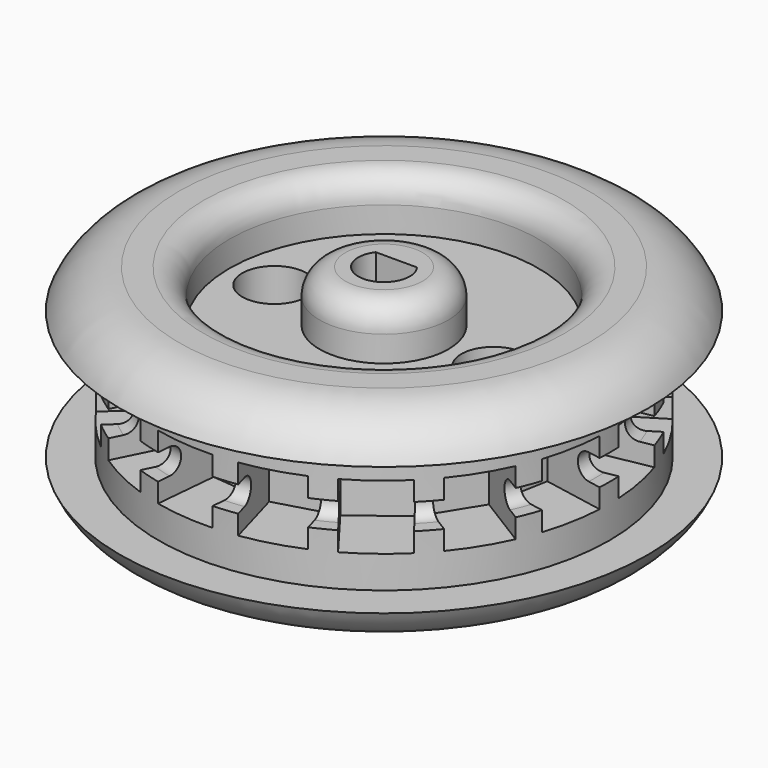
from build123d import *

# Parameters (mm, degrees)
F0_R      = 17.5
F1_DEPTH  = 10
F8_R      = 20.5
F8_R_2    = 17.5
F6_R      = 17.5
F9_DEPTH  = 3
F7_R      = 17.5
F10_R     = 20.5
F10_R_2   = 17.5
F11_DEPTH = 3
F14_DEPTH = 16.001
F15_R     = 4
F16_DEPTH = 5
F17_R     = 12
F17_R_2   = 8.5
F17_R_3   = 5
F18_DEPTH = 4
F19_R     = 2
F3_W      = 5
F3_H      = 4.6
F20_DEPTH = 2.5
F22_R     = 2.5
F23_DEPTH = 13


# Not quite as in the source:
# - a fillet or chamfer that OpenCascade refuses, or shapes differently, is made with other operations: its cross-section is extruded or revolved along the edge and cut away or added


with BuildPart() as f1:
    # F0 (on Top) → F1 (new body)
    with BuildSketch(Plane.XY):
        Circle(F0_R)
    extrude(amount=F1_DEPTH)

    # F8 (on face) + F6 (on face) → F9 (join)
    with BuildSketch(Plane.XY.offset(10)):
        Circle(F8_R)
        Circle(F8_R_2, mode=Mode.SUBTRACT)
    with BuildSketch(Plane.XY.offset(10)):
        Circle(F6_R)
    extrude(amount=F9_DEPTH)

    # F7 (on face) + F10 (on face) → F11 (join)
    with BuildSketch(Plane(origin=(0, 0, 0), x_dir=(1, 0, 0), z_dir=(0, 0, -1))):
        Circle(F7_R)
    with BuildSketch(Plane(origin=(0, 0, 0), x_dir=(1, 0, 0), z_dir=(0, 0, -1))):
        Circle(F10_R)
        Circle(F10_R_2, mode=Mode.SUBTRACT)
    extrude(amount=F11_DEPTH)

    # F12: fillet of radius 5 on 2 edges, made by hand

    # F12_s1 → F12_t2 (revolve, cut)
    with BuildSketch(Plane.XZ):
        with BuildLine():
            ThreePointArc((20.5, 0), (18.6560370926, -2.1833001327), (15.917424305, -3))
            Line((15.917424305, -3), (20.5, -3))
            Line((20.5, -3), (20.5, 0))
        make_face()
    revolve(axis=Axis((0, 0, -3), (0, 0, -1)), mode=Mode.SUBTRACT)

    # F12_s3 → F12_t4 (revolve, cut)
    with BuildSketch(Plane.XZ):
        with BuildLine():
            ThreePointArc((20.5, 10), (18.6560370926, 12.1833001327), (15.917424305, 13))
            Line((15.917424305, 13), (20.5, 13))
            Line((20.5, 13), (20.5, 10))
        make_face()
    revolve(axis=Axis((0, 0, 13), (0, 0, 1)), mode=Mode.SUBTRACT)

    # F13 (on face) → F14 (cut, through all)
    with BuildSketch(Plane.XY.offset(13)):
        with BuildLine():
            ThreePointArc((-1.6, 1.2), (-0.632455532, -1.8973665961), (2, 0))
            ThreePointArc((2, 0), (1.8973665961, 0.632455532), (1.6, 1.2))
            Line((1.6, 1.2), (-1.6, 1.2))
        make_face()
    extrude(amount=-F14_DEPTH, mode=Mode.SUBTRACT)

    # F15 (on face) → F16 (cut)
    with BuildSketch(Plane(origin=(0, 0, -3), x_dir=(1, 0, 0), z_dir=(0, 0, -1))):
        Circle(F15_R)
        with BuildLine():
            ThreePointArc((2, 0), (1.8973665961, -0.632455532), (1.6, -1.2))
            Line((1.6, -1.2), (-1.6, -1.2))
            ThreePointArc((-1.6, -1.2), (-0.632455532, 1.8973665961), (2, 0))
        make_face(mode=Mode.SUBTRACT)
    extrude(amount=-F16_DEPTH, mode=Mode.SUBTRACT)

    # F17 (on face) → F18 (cut)
    with BuildSketch(Plane.XY.offset(13)):
        Circle(F17_R)
        Circle(F17_R_2, mode=Mode.SUBTRACT)
        Circle(F17_R_2)
        Circle(F17_R_3, mode=Mode.SUBTRACT)
    extrude(amount=-F18_DEPTH, mode=Mode.SUBTRACT)

    # F19
    f19_edges = [f1.edges().sort_by_distance(p)[0] for p in [
        (-12, 0, 13),
        (-5, 0, 13),
    ]]
    fillet(f19_edges, radius=F19_R)

    # F3 (on offset) → F20 (cut, symmetric)
    with BuildSketch(Plane.XY.offset(5)):
        Polygon((-14.4821560317, -10.0899532542), (-11.383156071, -13.4893942734), (-7.6881114849, -10.1209160552), (-10.7871114456, -6.721475036), align=None)
        Polygon((-17.1491198468, -4.1770430306), (-15.4874081823, -8.4664152859), (-10.8250470353, -6.660206955), (-12.4867586998, -2.3708346997), align=None)
        with Locations((-15, 0)):
            Rectangle(F3_W, F3_H)
        Polygon((-15.4874081823, 8.4664152859), (-17.1491198468, 4.1770430306), (-12.4867586998, 2.3708346997), (-10.8250470353, 6.660206955), align=None)
        Polygon((-11.383156071, 13.4893942734), (-14.4821560317, 10.0899532542), (-10.7871114456, 6.721475036), (-7.6881114849, 10.1209160552), align=None)
        Polygon((-5.741545656, 16.690555817), (-9.8592967962, 14.6401593804), (-7.6306050173, 10.1643429237), (-3.5128538771, 12.2147393602), align=None)
        Polygon((0.6754923149, 17.6375653119), (-3.9048848961, 17.2131308584), (-3.4435430988, 12.2344599769), (1.1368341122, 12.6588944305), align=None)
        Polygon((7.0013013056, 16.2025238784), (2.576903347, 17.4613736327), (1.2085883966, 12.6522454168), (5.6329863552, 11.3933956625), align=None)
        Polygon((12.3815457594, 12.5792418137), (8.7106665139, 15.3513611411), (5.697493332, 11.3612750047), (9.3683725775, 8.5891556773), align=None)
        Polygon((16.0895938499, 7.2570634382), (13.6680059007, 11.1680622625), (9.416920222, 8.5359014481), (11.8385081712, 4.6249026238), align=None)
        Polygon((17.6246531354, 0.9547784325), (16.7794053535, 5.4764546911), (11.8645398551, 4.557707102), (12.709787637, 0.0360308434), align=None)
        Polygon((16.7794053535, -5.4764546911), (17.6246531354, -0.9547784325), (12.709787637, -0.0360308434), (11.8645398551, -4.557707102), align=None)
        Polygon((13.6680059007, -11.1680622625), (16.0895938499, -7.2570634382), (11.8385081712, -4.6249026238), (9.416920222, -8.5359014481), align=None)
        Polygon((8.7106665139, -15.3513611411), (12.3815457594, -12.5792418137), (9.3683725775, -8.5891556773), (5.697493332, -11.3612750047), align=None)
        Polygon((2.576903347, -17.4613736327), (7.0013013056, -16.2025238784), (5.6329863552, -11.3933956625), (1.2085883966, -12.6522454168), align=None)
        Polygon((-3.9048848961, -17.2131308584), (0.6754923149, -17.6375653119), (1.1368341122, -12.6588944305), (-3.4435430988, -12.2344599769), align=None)
        Polygon((-9.8592967962, -14.6401593804), (-5.741545656, -16.690555817), (-3.5128538771, -12.2147393602), (-7.6306050173, -10.1643429237), align=None)
    extrude(amount=F20_DEPTH, both=True, mode=Mode.SUBTRACT)

    # F5 (on Front) → F21 (revolve, cut)
    with BuildSketch(Plane.XZ):
        with BuildLine():
            Line((-17.5, 4), (-16.5, 4))
            ThreePointArc((-16.5, 4), (-15.5, 5), (-16.5, 6))
            Line((-16.5, 6), (-17.5, 6))
            Line((-17.5, 6), (-17.5, 4))
        make_face()
    revolve(axis=Axis((0, 0, 4.933624994), (0, 0, 1)), mode=Mode.SUBTRACT)

    # F22 (on face) → F23 (cut, through all)
    with BuildSketch(Plane.XY.offset(10)):
        with Locations((-8.5, 0)):
            Circle(F22_R)
        with Locations((8.5, 0)):
            Circle(F22_R)
    extrude(amount=-F23_DEPTH, mode=Mode.SUBTRACT)


solid = f1.part
